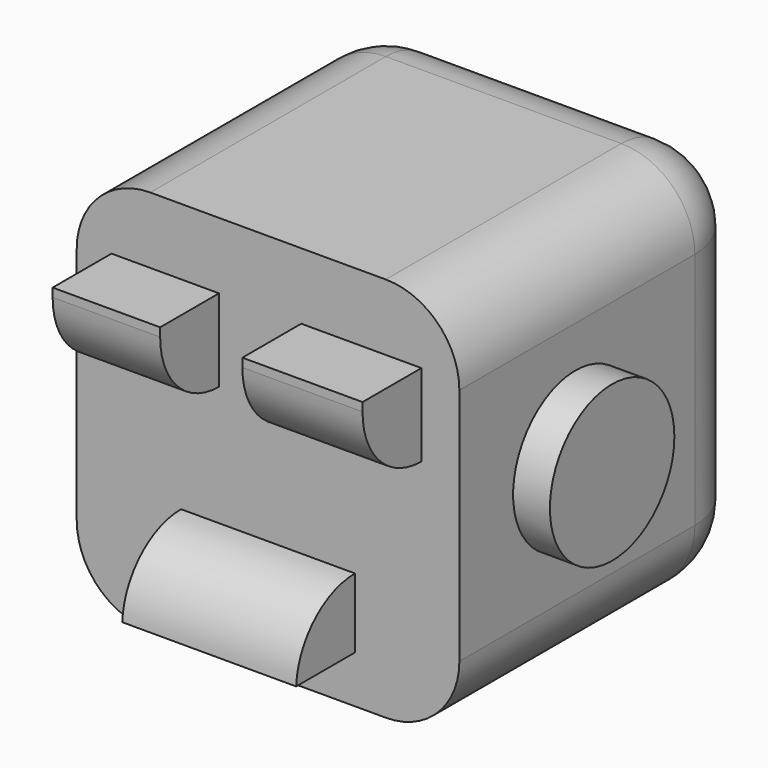
from build123d import *

# Parameters (mm, degrees)
F0_W        = 25.9993169457
F0_H        = 26.2141898274
F1_DEPTH    = 25
F2_R        = 5
F3_W        = 8.165073581
F3_H        = 5.5866301991
F3_W_2      = 7.3055946268
F4_W        = 11.8178697303
F4_H        = 4.7271503136
F5_DEPTH    = 5
F6_T1_DEPTH = 32.3055946268
F6_T3_DEPTH = 33.165073581
F6_T5_DEPTH = 36.7806185015
F7_R        = 5.2851135751
F9_DEPTH    = 2.5
F8_R        = 5.2456555176
F10_DEPTH   = 2.5
F11_R       = 5.0288488875
F12_DEPTH   = 5


# Not quite as in the source:
# - a fillet or chamfer that OpenCascade refuses, or shapes differently, is made with other operations: its cross-section is extruded or revolved along the edge and cut away or added


with BuildPart() as f1:
    # F0 (on Front) → F1 (new body)
    with BuildSketch(Plane.XZ):
        Rectangle(F0_W, F0_H)
    extrude(amount=F1_DEPTH)

    # F2
    f2_edges = [f1.edges().sort_by_distance(p)[0] for p in [
        (-12.999658, -12.5, 13.107095),
        (0, 0, 13.107095),
        (12.999658, -12.5, 13.107095),
        (12.999658, 0, 0),
        (12.999658, -12.5, -13.107095),
        (-12.999658, -12.5, -13.107095),
        (0, 0, -13.107095),
        (-12.999658, 0, 0),
    ]]
    fillet(f2_edges, radius=F2_R)

    # F3 (on face) + F4 (on face) → F5 (join)
    with BuildSketch(Plane.XZ.offset(25)):
        with Locations((6.3386769034, 5.8015007526)):
            Rectangle(F3_W, F3_H)
        with Locations((-6.9832885638, 5.8015007526)):
            Rectangle(F3_W_2, F3_H)
    with BuildSketch(Plane.XZ.offset(25)):
        with Locations((0, -7.5204637833)):
            Rectangle(F4_W, F4_H)
    extrude(amount=F5_DEPTH)

    # F6: fillet of radius 5 on 3 edges, made by hand

    # F6_s2 → F6_t1 (cut)
    with BuildSketch(Plane.YZ.offset(-23.1360858772)):
        with BuildLine():
            ThreePointArc((-25, 3.008185653), (-28.5355339059, 4.4726517471), (-30, 8.008185653))
            Line((-30, 8.008185653), (-30, 3.008185653))
            Line((-30, 3.008185653), (-25, 3.008185653))
        make_face()
    extrude(amount=F6_T1_DEPTH, mode=Mode.SUBTRACT)

    # F6_s4 → F6_t3 (cut)
    with BuildSketch(Plane.YZ.offset(-10.2438598871)):
        with BuildLine():
            ThreePointArc((-25, 3.008185653), (-28.5355339059, 4.4726517471), (-30, 8.008185653))
            Line((-30, 8.008185653), (-30, 3.008185653))
            Line((-30, 3.008185653), (-25, 3.008185653))
        make_face()
    extrude(amount=F6_T3_DEPTH, mode=Mode.SUBTRACT)

    # F6_s6 → F6_t5 (cut)
    with BuildSketch(Plane.YZ.offset(-18.3903092508)):
        with BuildLine():
            ThreePointArc((-25.0074502458, -5.1568886265), (-28.4451639895, -6.5261691088), (-30, -9.8840389401))
            Line((-30, -9.8840389401), (-30, -5.1568886265))
            Line((-30, -5.1568886265), (-25.0074502458, -5.1568886265))
        make_face()
    extrude(amount=F6_T5_DEPTH, mode=Mode.SUBTRACT)

    # F7 (on face) → F9 (join)
    with BuildSketch(Plane.YZ.offset(12.9996584728)):
        with Locations((-15.1483640075, 0)):
            Circle(F7_R)
    extrude(amount=F9_DEPTH)

    # F8 (on face) → F10 (join)
    with BuildSketch(Plane(origin=(-12.9996584728, 0, 0), x_dir=(0, -1, 0), z_dir=(-1, 0, 0))):
        with Locations((14.9334929883, 0)):
            Circle(F8_R)
    extrude(amount=F10_DEPTH)

    # F11 (on face) → F12 (cut)
    with BuildSketch(Plane(origin=(0, 0, -13.1070949137), x_dir=(1, 0, 0), z_dir=(0, 0, -1))):
        with Locations((0, 14.1341807321)):
            Circle(F11_R)
    extrude(amount=-F12_DEPTH, mode=Mode.SUBTRACT)


solid = f1.part
